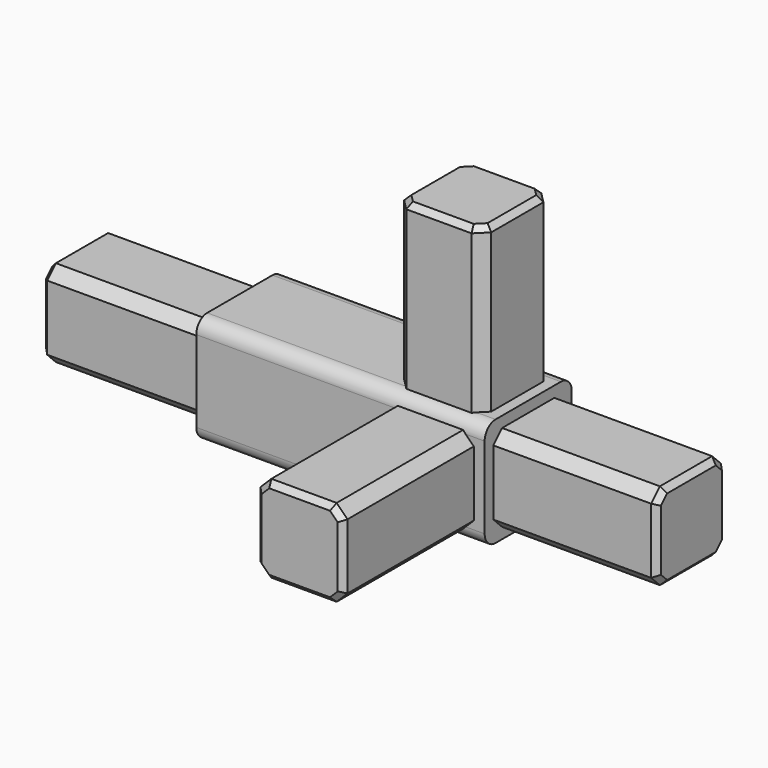
from build123d import *

# Parameters (mm, degrees)
F0_W          = 16
F0_H          = 16
F1_DEPTH      = 50
F0_W_2        = 20
F0_H_2        = 20
F2_DEPTH      = 20
F3_W          = 16
F3_H          = 16
F4_DEPTH      = 40
F5_W          = 16
F5_H          = 16
F6_DEPTH      = 73
F7_W          = 16
F7_H          = 16
F8_DEPTH      = 40
F9_DEPTH      = 33
F10_T1_DEPTH  = 65.5
F10_T6_DEPTH  = 65.5
F10_T11_DEPTH = 65.5
F10_T17_DEPTH = 65.5
F10_T22_DEPTH = 65.5
F10_T27_DEPTH = 65.5
F10_T32_DEPTH = 65.5
F10_T37_DEPTH = 65.5
F10_T42_DEPTH = 65.5
F10_T47_DEPTH = 65.5
F11_SIZE      = 2
F12_SIZE      = 1


# Not quite as in the source:
# - a fillet or chamfer that OpenCascade refuses, or shapes differently, is made with other operations: its cross-section is extruded or revolved along the edge and cut away or added


with BuildPart() as f1:
    # F0 (on Front) → F1 (new body)
    with BuildSketch(Plane.XZ):
        Rectangle(F0_W, F0_H)
    extrude(amount=F1_DEPTH)

    # F0 (on Front) → F2 (join)
    with BuildSketch(Plane.XZ):
        Rectangle(F0_W_2, F0_H_2)
        Rectangle(F0_W, F0_H, mode=Mode.SUBTRACT)
    extrude(amount=F2_DEPTH)

    # F3 (on Right) → F4 (join)
    with BuildSketch(Plane.YZ):
        with Locations((-10, 0)):
            Rectangle(F3_W, F3_H)
    extrude(amount=F4_DEPTH)

    # F5 (on Right) → F6 (join)
    with BuildSketch(Plane.YZ):
        with Locations((-10, 0)):
            Rectangle(F5_W, F5_H)
    extrude(amount=-F6_DEPTH)

    # F7 (on Top) → F8 (join)
    with BuildSketch(Plane.XY):
        with Locations((0, -10)):
            Rectangle(F7_W, F7_H)
    extrude(amount=F8_DEPTH)

    # F9 (add): a face of the model
    f9_faces = [f1.faces().sort_by_distance(p)[0] for p in [
        (-10, -10, 9.7171572875),
    ]]
    extrude(f9_faces, amount=F9_DEPTH)

    # F10: fillet of radius 2.5 on 4 edges, made by hand

    # F10_s2 → F10_t1 (cut)
    with BuildSketch(Plane.YZ.offset(-49.25)):
        with BuildLine():
            ThreePointArc((-2.5, -10), (-0.732233047, -9.267766953), (0, -7.5))
            Line((0, -7.5), (0, -10))
            Line((0, -10), (-2.5, -10))
        make_face()
    extrude(amount=F10_T1_DEPTH, mode=Mode.SUBTRACT)


with BuildPart() as f10_tool4:
    # F10_s5 → F10_t6 (new body)
    with BuildSketch(Plane.YZ.offset(16.25)):
        with BuildLine():
            ThreePointArc((-20, 7.5), (-19.267766953, 9.267766953), (-17.5, 10))
            Line((-17.5, 10), (-20, 10))
            Line((-20, 10), (-20, 7.5))
        make_face()
    extrude(amount=-F10_T6_DEPTH)

    split(bisect_by=Plane.YZ.offset(8), keep=Keep.TOP)


with BuildPart() as f1_1:
    add(f1.part)

    # F10_t3: cut F10_tool4
    add(f10_tool4.part, mode=Mode.SUBTRACT)


with BuildPart() as f10_tool9:
    # F10_s10 → F10_t11 (new body)
    with BuildSketch(Plane.YZ.offset(16.25)):
        with BuildLine():
            ThreePointArc((-20, 7.5), (-19.267766953, 9.267766953), (-17.5, 10))
            Line((-17.5, 10), (-20, 10))
            Line((-20, 10), (-20, 7.5))
        make_face()
    extrude(amount=-F10_T11_DEPTH)

    split(bisect_by=Plane.XY.offset(8), keep=Keep.TOP)

    split(bisect_by=Plane.XZ.offset(18), keep=Keep.TOP)


with BuildPart() as f1_2:
    add(f1_1.part)

    # F10_t8: cut F10_tool9
    add(f10_tool9.part, mode=Mode.SUBTRACT)


with BuildPart() as f10_tool15:
    # F10_s16 → F10_t17 (new body)
    with BuildSketch(Plane.YZ.offset(16.25)):
        with BuildLine():
            ThreePointArc((-20, 7.5), (-19.267766953, 9.267766953), (-17.5, 10))
            Line((-17.5, 10), (-20, 10))
            Line((-20, 10), (-20, 7.5))
        make_face()
    extrude(amount=-F10_T17_DEPTH)

    split(bisect_by=Plane.YZ.offset(-8), keep=Keep.BOTTOM)


with BuildPart() as f1_3:
    add(f1_2.part)

    # F10_t14: cut F10_tool15
    add(f10_tool15.part, mode=Mode.SUBTRACT)


with BuildPart() as f10_tool20:
    # F10_s21 → F10_t22 (new body)
    with BuildSketch(Plane.YZ.offset(-49.25)):
        with BuildLine():
            ThreePointArc((-20, -7.5), (-19.267766953, -9.267766953), (-17.5, -10))
            Line((-17.5, -10), (-20, -10))
            Line((-20, -10), (-20, -7.5))
        make_face()
    extrude(amount=F10_T22_DEPTH)

    split(bisect_by=Plane.YZ.offset(-8), keep=Keep.BOTTOM)


with BuildPart() as f1_4:
    add(f1_3.part)

    # F10_t19: cut F10_tool20
    add(f10_tool20.part, mode=Mode.SUBTRACT)


with BuildPart() as f10_tool25:
    # F10_s26 → F10_t27 (new body)
    with BuildSketch(Plane.YZ.offset(-49.25)):
        with BuildLine():
            ThreePointArc((-20, -7.5), (-19.267766953, -9.267766953), (-17.5, -10))
            Line((-17.5, -10), (-20, -10))
            Line((-20, -10), (-20, -7.5))
        make_face()
    extrude(amount=F10_T27_DEPTH)

    split(bisect_by=Plane.XY.offset(-8), keep=Keep.BOTTOM)


with BuildPart() as f1_5:
    add(f1_4.part)

    # F10_t24: cut F10_tool25
    add(f10_tool25.part, mode=Mode.SUBTRACT)


with BuildPart() as f10_tool30:
    # F10_s31 → F10_t32 (new body)
    with BuildSketch(Plane.YZ.offset(-49.25)):
        with BuildLine():
            ThreePointArc((-20, -7.5), (-19.267766953, -9.267766953), (-17.5, -10))
            Line((-17.5, -10), (-20, -10))
            Line((-20, -10), (-20, -7.5))
        make_face()
    extrude(amount=F10_T32_DEPTH)

    split(bisect_by=Plane.YZ.offset(8), keep=Keep.TOP)


with BuildPart() as f1_6:
    add(f1_5.part)

    # F10_t29: cut F10_tool30
    add(f10_tool30.part, mode=Mode.SUBTRACT)


with BuildPart() as f10_tool35:
    # F10_s36 → F10_t37 (new body)
    with BuildSketch(Plane.YZ.offset(16.25)):
        with BuildLine():
            ThreePointArc((0, 7.5), (-0.732233047, 9.267766953), (-2.5, 10))
            Line((-2.5, 10), (0, 10))
            Line((0, 10), (0, 7.5))
        make_face()
    extrude(amount=-F10_T37_DEPTH)

    split(bisect_by=Plane.XZ.offset(2), keep=Keep.BOTTOM)


with BuildPart() as f1_7:
    add(f1_6.part)

    # F10_t34: cut F10_tool35
    add(f10_tool35.part, mode=Mode.SUBTRACT)


with BuildPart() as f10_tool40:
    # F10_s41 → F10_t42 (new body)
    with BuildSketch(Plane.YZ.offset(16.25)):
        with BuildLine():
            ThreePointArc((0, 7.5), (-0.732233047, 9.267766953), (-2.5, 10))
            Line((-2.5, 10), (0, 10))
            Line((0, 10), (0, 7.5))
        make_face()
    extrude(amount=-F10_T42_DEPTH)

    split(bisect_by=Plane.YZ.offset(8), keep=Keep.TOP)


with BuildPart() as f1_8:
    add(f1_7.part)

    # F10_t39: cut F10_tool40
    add(f10_tool40.part, mode=Mode.SUBTRACT)


with BuildPart() as f10_tool45:
    # F10_s46 → F10_t47 (new body)
    with BuildSketch(Plane.YZ.offset(16.25)):
        with BuildLine():
            ThreePointArc((0, 7.5), (-0.732233047, 9.267766953), (-2.5, 10))
            Line((-2.5, 10), (0, 10))
            Line((0, 10), (0, 7.5))
        make_face()
    extrude(amount=-F10_T47_DEPTH)

    split(bisect_by=Plane.YZ.offset(-8), keep=Keep.BOTTOM)


with BuildPart() as f1_9:
    add(f1_8.part)

    # F10_t44: cut F10_tool45
    add(f10_tool45.part, mode=Mode.SUBTRACT)

    # F11
    f11_edges = [f1_9.edges().sort_by_distance(p)[0] for p in [
        (-58, -18, 8),
        (-58, -18, -8),
        (-58, -2, 8),
        (-58, -2, -8),
        (-8, -34.974745, 8),
        (-8, -34.974745, -8),
        (8, -34.974745, 8),
        (8, -34.974745, -8),
        (25, -18, -8),
        (25, -18, 8),
        (8, -18, 24.974745),
        (-8, -18, 24.974745),
        (25, -2, -8),
        (25, -2, 8),
        (8, -2, 24.974745),
        (-8, -2, 24.974745),
    ]]
    chamfer(f11_edges, length=F11_SIZE)

    # F12
    f12_edges = [f1_9.edges().sort_by_distance(p)[0] for p in [
        (-73, -10, 8),
        (-73, -10, -8),
        (-73, -17, -7),
        (-73, -3, -7),
        (-73, -18, 0),
        (-73, -2, 0),
        (-73, -17, 7),
        (-73, -3, 7),
        (-8, -50, 0),
        (-7, -50, 7),
        (-7, -50, -7),
        (0, -50, 8),
        (0, -50, -8),
        (7, -50, 7),
        (7, -50, -7),
        (8, -50, 0),
        (-8, -10, 40),
        (-7, -3, 40),
        (-7, -17, 40),
        (0, -2, 40),
        (0, -18, 40),
        (7, -3, 40),
        (7, -17, 40),
        (8, -10, 40),
        (40, -10, -8),
        (40, -17, -7),
        (40, -3, -7),
        (40, -18, 0),
        (40, -2, 0),
        (40, -17, 7),
        (40, -3, 7),
        (40, -10, 8),
    ]]
    chamfer(f12_edges, length=F12_SIZE)


solid = f1_9.part
